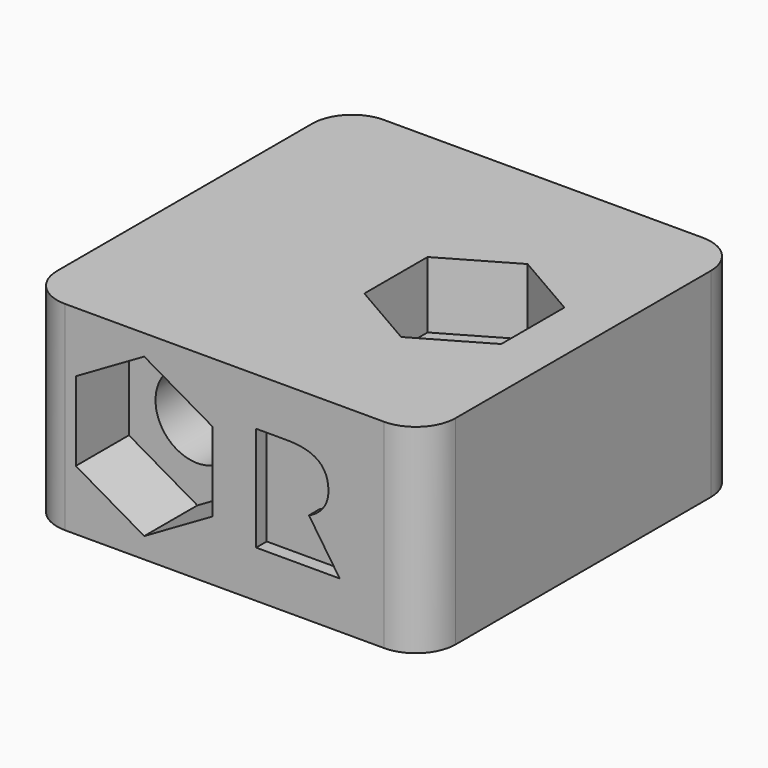
from build123d import *

# Parameters (mm, degrees)
F2_W          = 30
F2_H          = 30
F2_R          = 3.15
F3_DEPTH      = 7.5
F4_R          = 3.15
F5_DEPTH      = 30
F7_R          = 3
F8_DEPTH      = 5
F6_R          = 3.15
F9_DEPTH      = 5
F10_TEXT_SIZE = 11.0344827586
F11_DEPTH     = 1


# Not quite as in the source:
# - Text() gives the source's letters only with a copy of the font that has no kerning and outlines rounded to 1/6400 em; it was checked with that copy


with BuildPart() as f3:
    # F2 (on Top) → F3 (new body, symmetric)
    with BuildSketch(Plane.XY):
        Rectangle(F2_W, F2_H)
        with Locations((6.05, 0)):
            Circle(F2_R, mode=Mode.SUBTRACT)
    extrude(amount=F3_DEPTH, both=True)

    # F4 (on face) → F5 (cut, through all)
    with BuildSketch(Plane.XZ.offset(15)):
        with Locations((-6.05, 0)):
            Circle(F4_R)
    extrude(amount=-F5_DEPTH, mode=Mode.SUBTRACT)

    # F7
    f7_edges = [f3.edges().sort_by_distance(p)[0] for p in [
        (-15, -15, 0),
        (15, -15, 0),
        (15, 15, 0),
        (-15, 15, 0),
    ]]
    fillet(f7_edges, radius=F7_R)

    # F4 (on face) → F8 (cut)
    with BuildSketch(Plane.XZ.offset(15)):
        Polygon((-6.05, -5.9467077727), (-0.9, -2.9733538863), (-0.9, 2.9733538863), (-6.05, 5.9467077727), (-11.2, 2.9733538863), (-11.2, -2.9733538863), align=None)
        with Locations((-6.05, 0)):
            Circle(F4_R, mode=Mode.SUBTRACT)
    extrude(amount=-F8_DEPTH, mode=Mode.SUBTRACT)

    # F6 (on face) → F9 (cut)
    with BuildSketch(Plane.XY.offset(7.5)):
        Polygon((6.05, -5.9467077727), (11.2, -2.9733538863), (11.2, 2.9733538863), (6.05, 5.9467077727), (0.9, 2.9733538863), (0.9, -2.9733538863), align=None)
        with Locations((6.05, 0)):
            Circle(F6_R, mode=Mode.SUBTRACT)
    extrude(amount=-F9_DEPTH, mode=Mode.SUBTRACT)

    # F10 (on face) → F11 (cut)
    with BuildSketch(Plane.XZ.offset(15)):
        with Locations((1.3824919225, -3.9724137931)):
            Text('R', F10_TEXT_SIZE, font='Open Sans', font_style=FontStyle.BOLD, text_align=(TextAlign.LEFT, TextAlign.BOTTOM))
        Polygon((4.044560888, -0.95), (4.044560888, -3.9724137931), (6.8135264053, -3.9724137931), (4.9324919225, -0.95), align=None)
        with BuildLine():
            Line((4.044560888, 2.5362068966), (4.044560888, 0.4086206897))
            Line((4.044560888, 0.4086206897), (4.5824919225, 0.4086206897))
            add(Edge.make_bspline(
                [(4.5824919225, 0.4086206897), (5.3755953708, 0.4086206897), (5.7523195087, 0.6724137931)],
                knots=[0, 0, 0, 1, 1, 1], degree=2))
            add(Edge.make_bspline(
                [(5.7523195087, 0.6724137931), (6.1290436466, 0.9362068966), (6.1290436466, 1.5017241379)],
                knots=[0, 0, 0, 1, 1, 1], degree=2))
            add(Edge.make_bspline(
                [(6.1290436466, 1.5017241379), (6.1290436466, 2.0620689655), (5.743698819, 2.299137931)],
                knots=[0, 0, 0, 1, 1, 1], degree=2))
            add(Edge.make_bspline(
                [(5.743698819, 2.299137931), (5.3583539915, 2.5362068966), (4.5514574397, 2.5362068966)],
                knots=[0, 0, 0, 1, 1, 1], degree=2))
            Line((4.5514574397, 2.5362068966), (4.044560888, 2.5362068966))
        make_face()
    extrude(amount=-F11_DEPTH, mode=Mode.SUBTRACT)


solid = f3.part
